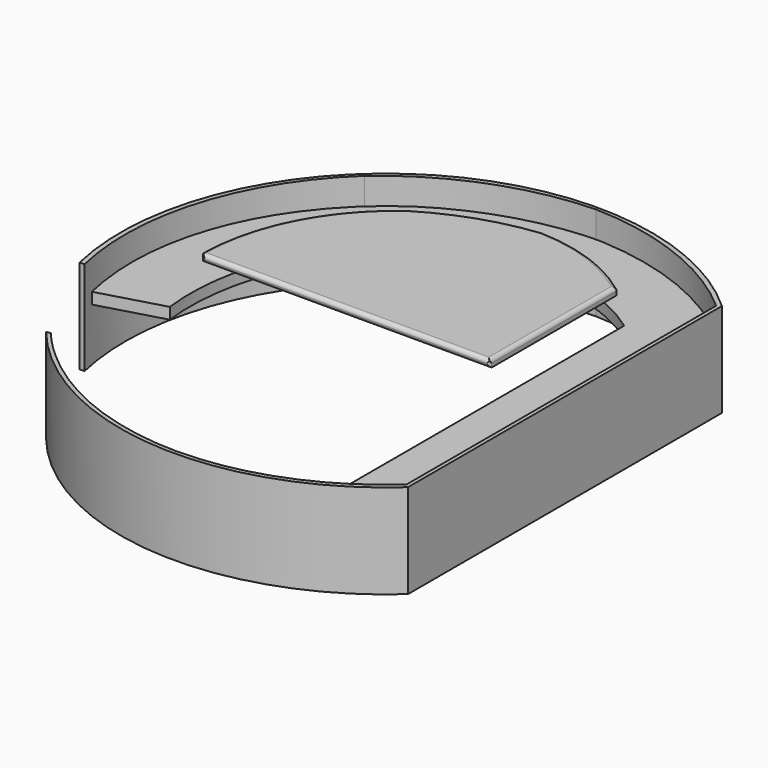
from build123d import *

# Parameters (mm, degrees)
F1_DEPTH     = 25
F4_DEPTH     = 3
F7_DEPTH     = 2
F8_T1_DEPTH  = 46.5490327792
F8_T3_DEPTH  = 79.7769061223
F8_T6_ANGLE  = 57.5412120426
F8_T8_ANGLE  = 53.8676992582
F8_T10_ANGLE = 42.3774462238


# Not quite as in the source:
# - a fillet or chamfer that OpenCascade refuses, or shapes differently, is made with other operations: its cross-section is extruded or revolved along the edge and cut away or added


with BuildPart() as f1:
    # F0 (on Top) → F1 (new body)
    with BuildSketch(Plane.XY):
        with BuildLine():
            Line((-53.5594895482, -44.3499796093), (-54.6605306502, -44.5250085798))
            ThreePointArc((-54.6605306502, -44.5250085798), (-5.2104245552, -70.3071936288), (47.5, -52.0960651105))
            Line((47.5, -52.0960651105), (47.5, 52.0960651105))
            ThreePointArc((47.5, 52.0960651105), (-35.5788922727, 60.863720102), (-68.6997002997, -15.8303878265))
            Line((-68.6997002997, -15.8303878265), (-67.4245581031, -15.8242937177))
            ThreePointArc((-67.4245581031, -15.8242937177), (-66.1215536717, 20.5568874041), (-46.8615852296, 51.4493100345))
            ThreePointArc((-46.8615852296, 51.4493100345), (-24.9971695074, 64.5844738855), (0, 69.6566253901))
            ThreePointArc((0, 69.6566253901), (24.8405659763, 64.6202381597), (46.4957170188, 51.4493100345))
            Line((46.4957170188, 51.4493100345), (46.4957170188, -51.2676276267))
            ThreePointArc((46.4957170188, -51.2676276267), (24.9448717462, -64.7072512948), (0, -69.4838389754))
            ThreePointArc((0, -69.4838389754), (-25.111447228, -64.6992524943), (-46.8615852296, -51.2676276267))
            ThreePointArc((-46.8615852296, -51.2676276267), (-50.3311740259, -47.9256081518), (-53.5594895482, -44.3499796093))
        make_face()
    extrude(amount=F1_DEPTH)

    # F3 (on offset) → F4 (join)
    with BuildSketch(Plane.XY.offset(18)):
        with BuildLine():
            ThreePointArc((-50.0496417258, -9.2208846097), (-50.2644885848, 3.5139765926), (-47.8203118252, 16.0139305517))
            ThreePointArc((-47.8203118252, 16.0139305517), (-42.0194626362, 28.096227029), (-34.1098720099, 38.9161214649))
            ThreePointArc((-34.1098720099, 38.9161214649), (-24.6335675904, 45.6735792578), (-13.8310398906, 50.0058969483))
            ThreePointArc((-13.8310398906, 50.0058969483), (-6.8813374216, 51.9550402589), (0.3012418747, 52.6678366587))
            ThreePointArc((0.3012418747, 52.6678366587), (15.2727192247, 49.9993037861), (28.7969588935, 43.0450861367))
            Line((28.7969588935, 43.0450861367), (28.7969588935, -62.2076252475))
            ThreePointArc((28.7969588935, -62.2076252475), (38.2157263655, -57.1420397054), (46.7044785619, -50.6370859221))
            Line((46.7044785619, -50.6370859221), (46.7044785619, 51.9938943908))
            ThreePointArc((46.7044785619, 51.9938943908), (-6.9617735399, 69.2076002087), (-55.7927936316, 41.0667089745))
            ThreePointArc((-55.7927936316, 41.0667089745), (-65.337409162, 22.6733320453), (-68.737745285, 2.2318615811))
            ThreePointArc((-68.737745285, 2.2318615811), (-68.3088903863, -5.9408679833), (-66.9282525778, -14.007544145))
            Line((-66.9282525778, -14.007544145), (-50.0496417258, -9.2208846097))
        make_face()
    extrude(amount=-F4_DEPTH)


with BuildPart() as f7:
    # F6 (on offset) → F7 (new body)
    with BuildSketch(Plane.XY.offset(25)):
        with BuildLine():
            ThreePointArc((0, 51.9124306738), (-14.7201548314, 48.6195532067), (-28.3503979445, 42.1587117016))
            ThreePointArc((-28.3503979445, 42.1587117016), (-43.6028608691, 24.2823909868), (-49.4652068528, 1.5264386417))
            ThreePointArc((-49.4652068528, 1.5264386417), (-48.9688767374, 0.5048791333), (-47.951515212, 0))
            Line((-47.951515212, 0), (26.8253909103, 0))
            ThreePointArc((26.8253909103, 0), (27.2387043365, 0.2132332003), (27.4818651378, 0.6096789225))
            Line((27.4818651378, 0.6096789225), (27.4818651378, 42.1587117016))
            ThreePointArc((27.4818651378, 42.1587117016), (14.5082557431, 49.1975641723), (0, 51.9124306738))
        make_face()
    extrude(amount=F7_DEPTH)

    # F8: fillet of radius 1 on 6 edges, made by hand

    # F8_s2 → F8_t1 (cut)
    with BuildSketch(Plane.XZ.offset(-44.6587117016)):
        with BuildLine():
            ThreePointArc((27.4818651378, 26), (27.188971919, 26.7071067812), (26.4818651378, 27))
            Line((26.4818651378, 27), (27.4818651378, 27))
            Line((27.4818651378, 27), (27.4818651378, 26))
        make_face()
    extrude(amount=F8_T1_DEPTH, mode=Mode.SUBTRACT)

    # F8_s4 → F8_t3 (cut)
    with BuildSketch(Plane.YZ.offset(-50.451515212)):
        with BuildLine():
            ThreePointArc((0, 26), (0.2928932188, 26.7071067812), (1, 27))
            Line((1, 27), (0, 27))
            Line((0, 27), (0, 26))
        make_face()
        with BuildLine():
            ThreePointArc((0, 26), (0.2928932188, 25.2928932188), (1, 25))
            Line((1, 25), (0, 25))
            Line((0, 25), (0, 26))
        make_face()
    extrude(amount=F8_T3_DEPTH, mode=Mode.SUBTRACT)

    # F8_s5 → F8_t6 (revolve, cut)
    with BuildSketch(Plane(origin=(1.9677553856, 1.3158294554, 0), x_dir=(0, 0, 1), z_dir=(0.8312710302, 0.5558673172, 0))):
        with BuildLine():
            ThreePointArc((26, -50.8642670989), (26.7071067812, -50.5713738801), (27, -49.8642670989))
            Line((27, -49.8642670989), (27, -50.8642670989))
            Line((27, -50.8642670989), (26, -50.8642670989))
        make_face()
    revolve(axis=Axis((2.6999679754, 0.2208431249, 27), (0, 0, 1)), revolution_arc=F8_T6_ANGLE, mode=Mode.SUBTRACT)

    # F8_s7 → F8_t8 (revolve, cut)
    with BuildSketch(Plane(origin=(-2.9923866857, 2.5503787428, 0), x_dir=(0, 0, 1), z_dir=(0.7610789086, -0.6486593057, 0))):
        with BuildLine():
            ThreePointArc((26, -49.9782811264), (26.7071067812, -49.6853879076), (27, -48.9782811264))
            Line((27, -48.9782811264), (27, -49.9782811264))
            Line((27, -49.9782811264), (26, -49.9782811264))
        make_face()
    revolve(axis=Axis((-1.3732816064, 4.4500920681, 27), (0, 0, 1)), revolution_arc=F8_T8_ANGLE, mode=Mode.SUBTRACT)

    # F8_s9 → F8_t10 (revolve, cut)
    with BuildSketch(Plane(origin=(7.3996724265, -0.0121620406, 0), x_dir=(0, 0, 1), z_dir=(0.9999986493, -0.0016435895, 0))):
        with BuildLine():
            ThreePointArc((26, -52.3260934279), (26.7071067812, -52.0332002091), (27, -51.3260934279))
            Line((27, -51.3260934279), (27, -52.3260934279))
            Line((27, -52.3260934279), (26, -52.3260934279))
        make_face()
    revolve(axis=Axis((7.374052369, -15.600009422, 27), (0, 0, 1)), revolution_arc=F8_T10_ANGLE, mode=Mode.SUBTRACT)


solid = Compound([f1.part, f7.part])
